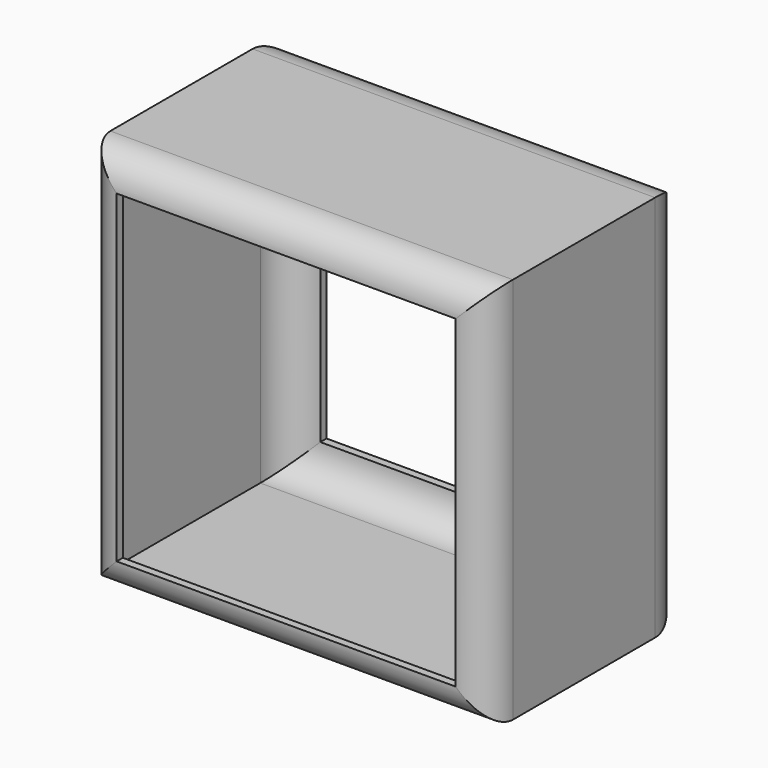
from build123d import *

# Parameters (mm, degrees)
F0_W     = 132.177695632
F0_H     = 127.1953880787
F1_DEPTH = 82.296
F2_R     = 10.4245741623
F3_R     = 13.4906253865
F4_T     = -2.54


# Not quite as in the source:
# - a shell that OpenCascade refuses in one call is made with other operations: the cavity is built on its own and cut out


with BuildPart() as f1:
    # F0 (on Front) → F1 (new body)
    with BuildSketch(Plane.XZ):
        with Locations((2.9307678342, -2.1980777383)):
            Rectangle(F0_W, F0_H)
    extrude(amount=F1_DEPTH)

    # F2
    f2_edges = [f1.edges().sort_by_distance(p)[0] for p in [
        (2.930768, -82.296, 61.399616),
        (-63.15808, -82.296, -2.198078),
        (2.930768, -82.296, -65.795772),
        (69.019616, -82.296, -2.198078),
    ]]
    fillet(f2_edges, radius=F2_R)

    # F3
    f3_edges = [f1.edges().sort_by_distance(p)[0] for p in [
        (2.930768, 0, 61.399616),
        (-63.15808, 0, -2.198078),
        (2.930768, 0, -65.795772),
        (69.019616, 0, -2.198078),
    ]]
    fillet(f3_edges, radius=F3_R)

    # F4: a shell. OpenCascade refuses it in one call, so the cavity is built on its own and cut out:
    # the body offset inwards by the wall thickness, plus a prism from it out through each open face.
    f4_core = offset(f1.part, amount=F4_T, mode=Mode.PRIVATE)
    f4_exits = [f4_core.faces().sort_by_distance(p)[0] for p in [
        (2.930768, -79.756, -2.198078),
        (2.930768, -2.54, -2.198078),
    ]]
    add(f4_core, mode=Mode.SUBTRACT)
    extrude(f4_exits, amount=-F4_T, mode=Mode.SUBTRACT)


solid = f1.part
